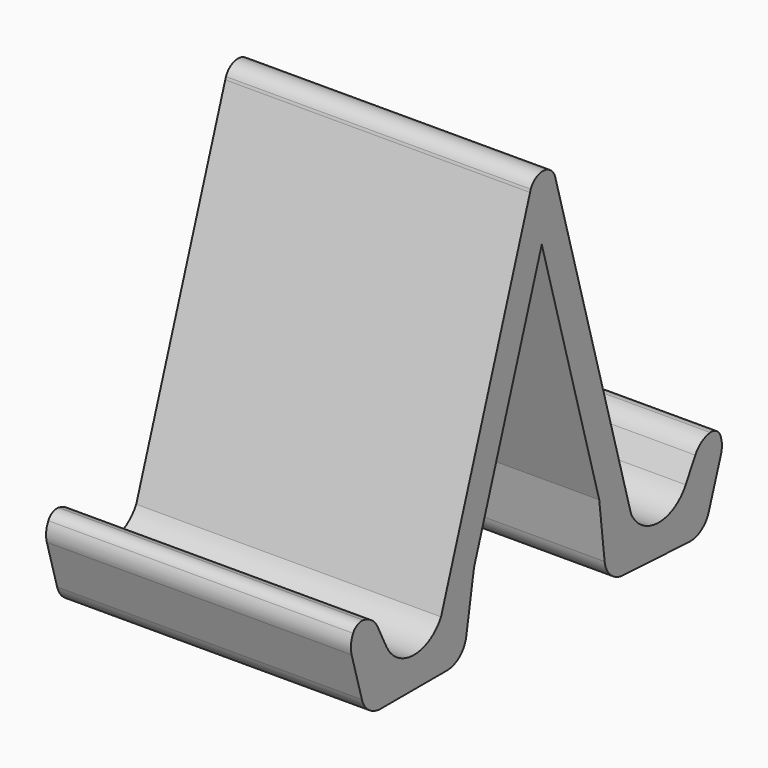
from build123d import *

# Parameters (mm, degrees)
F1_DEPTH    = 25
F2_T1_DEPTH = 35
F2_T3_DEPTH = 33.3163528131
F3_R        = 1
F4_R        = 2


# Not quite as in the source:
# - a fillet or chamfer that OpenCascade refuses, or shapes differently, is made with other operations: its cross-section is extruded or revolved along the edge and cut away or added


with BuildPart() as f1:
    # F0 (on Right) → F1 (new body)
    with BuildSketch(Plane.YZ):
        with BuildLine():
            Line((-6.9323359057, 13.8083724305), (-5, 7.0966093383))
            Line((-5, 7.0966093383), (-0.1434815237, 7.0966093383))
            ThreePointArc((-0.1434815237, 7.0966093383), (-3.0832893136, 7.9619770163), (-5.1434815237, 10.2306636665))
            Line((-5.1434815237, 10.2306636665), (-6.9323359057, 13.8083724305))
        make_face()
        with BuildLine():
            ThreePointArc((-5.1434815237, 10.2306636665), (-3.0832893136, 7.9619770163), (-0.1434815237, 7.0966093383))
            Line((-0.1434815237, 7.0966093383), (0, 7.0966093383))
            ThreePointArc((0, 7.0966093383), (2.9398077898, 7.9619770163), (5, 10.2306636665))
            Line((5, 10.2306636665), (6.0755903162, 13.4044619593))
            Line((6.0755903162, 13.4044619593), (13.0241518458, 33.9079309741))
            Line((13.0241518458, 33.9079309741), (11.8234508953, 38.1539476614))
            Line((11.8234508953, 38.1539476614), (2.6952738362, 11.2189777838))
            ThreePointArc((2.6952738362, 11.2189777838), (-0.1451253509, 9.597004922), (-2.9074135462, 11.3486976553))
            Line((-2.9074135462, 11.3486976553), (-4.6962679282, 14.9264064193))
            Line((-4.6962679282, 14.9264064193), (-6.9323359057, 13.8083724305))
            Line((-6.9323359057, 13.8083724305), (-5.1434815237, 10.2306636665))
        make_face()
        with BuildLine():
            ThreePointArc((5, 10.2306636665), (2.9398077898, 7.9619770163), (0, 7.0966093383))
            Line((0, 7.0966093383), (5, 7.0966093383))
            Line((5, 7.0966093383), (6.0755903162, 13.4044619593))
            Line((6.0755903162, 13.4044619593), (5, 10.2306636665))
        make_face()
        with BuildLine():
            Line((11.8234508953, 38.1539476614), (13.0241518458, 33.9079309741))
            Line((13.0241518458, 33.9079309741), (14.4404213471, 38.0869884254))
            Line((14.4404213471, 38.0869884254), (14.3799488187, 38.3008363155))
            ThreePointArc((14.3799488187, 38.3008363155), (13.1588056017, 39.1706090028), (11.8947803947, 38.3644231928))
            Line((11.8947803947, 38.3644231928), (11.8234508953, 38.1539476614))
        make_face()
        with BuildLine():
            Line((14.4404213471, 38.0869884254), (13.0241518458, 33.9079309741))
            Line((13.0241518458, 33.9079309741), (18.9150818034, 13.075943714))
            Line((18.9150818034, 13.075943714), (19.8269579074, 9.8512930193))
            ThreePointArc((19.8269579074, 9.8512930193), (21.7684346268, 7.4802174812), (24.6601411506, 6.4656414912))
            Line((24.6601411506, 6.4656414912), (24.8034349308, 6.4583039016))
            ThreePointArc((24.8034349308, 6.4583039016), (27.7836505914, 7.1721986247), (29.9571668266, 9.332559297))
            Line((29.9571668266, 9.332559297), (31.9266431601, 12.8141053576))
            Line((31.9266431601, 12.8141053576), (29.7506768723, 14.045028066))
            Line((29.7506768723, 14.045028066), (27.7812005388, 10.5634820055))
            ThreePointArc((27.7812005388, 10.5634820055), (24.9329458702, 8.9553436878), (22.1792103708, 10.7204511366))
            Line((22.1792103708, 10.7204511366), (14.4404213471, 38.0869884254))
        make_face()
        with BuildLine():
            Line((19.8269579074, 9.8512930193), (18.9150818034, 13.075943714))
            Line((18.9150818034, 13.075943714), (19.6666835811, 6.7213395575))
            Line((19.6666835811, 6.7213395575), (24.6601411506, 6.4656414912))
            ThreePointArc((24.6601411506, 6.4656414912), (21.7684346268, 7.4802174812), (19.8269579074, 9.8512930193))
        make_face()
        with BuildLine():
            ThreePointArc((29.9571668266, 9.332559297), (27.7836505914, 7.1721986247), (24.8034349308, 6.4583039016))
            Line((24.8034349308, 6.4583039016), (29.6535987202, 6.2099434249))
            Line((29.6535987202, 6.2099434249), (31.9266431601, 12.8141053576))
            Line((31.9266431601, 12.8141053576), (29.9571668266, 9.332559297))
        make_face()
    extrude(amount=F1_DEPTH)

    # F2: fillet of radius 2 on 4 edges, made by hand

    # F2_s2 → F2_t1 (cut)
    with BuildSketch(Plane.YZ.offset(-5)):
        with BuildLine():
            ThreePointArc((-3.8018407372, 13.1375520373), (-4.9582395872, 14.1404914424), (-6.4851223102, 14.0319792283))
            Line((-6.4851223102, 14.0319792283), (-4.6962679282, 14.9264064193))
            Line((-4.6962679282, 14.9264064193), (-3.8018407372, 13.1375520373))
        make_face()
        with BuildLine():
            ThreePointArc((31.4914499025, 13.0602898993), (29.972114357, 13.2467443186), (28.7659387055, 12.3042550357))
            Line((28.7659387055, 12.3042550357), (29.7506768723, 14.045028066))
            Line((29.7506768723, 14.045028066), (31.4914499025, 13.0602898993))
        make_face()
    extrude(amount=F2_T1_DEPTH, mode=Mode.SUBTRACT)

    # F2_s4 → F2_t3 (cut)
    with BuildSketch(Plane.YZ.offset(-4.1581764065)):
        with BuildLine():
            ThreePointArc((-6.4721671557, 12.2100252573), (-6.3817440303, 13.5668302715), (-5.4446614885, 14.5522096391))
            Line((-5.4446614885, 14.5522096391), (-6.9323359057, 13.8083724305))
            Line((-6.9323359057, 13.8083724305), (-6.4721671557, 12.2100252573))
        make_face()
        with BuildLine():
            ThreePointArc((31.3853376782, 11.2413824514), (31.3644193539, 12.6010363088), (30.4789548914, 13.6330483599))
            Line((30.4789548914, 13.6330483599), (31.9266431601, 12.8141053576))
            Line((31.9266431601, 12.8141053576), (31.3853376782, 11.2413824514))
        make_face()
    extrude(amount=F2_T3_DEPTH, mode=Mode.SUBTRACT)

    # F3
    f3_edges = [f1.edges().sort_by_distance(p)[0] for p in [
        (12.5, -5.926233, 14.214777),
        (12.5, 30.942641, 13.27143),
    ]]
    fillet(f3_edges, radius=F3_R)

    # F4
    f4_edges = [f1.edges().sort_by_distance(p)[0] for p in [
        (12.5, -5, 7.096609),
        (12.5, 5, 7.096609),
        (12.5, 19.666684, 6.72134),
        (12.5, 29.653599, 6.209943),
    ]]
    fillet(f4_edges, radius=F4_R)


solid = f1.part
